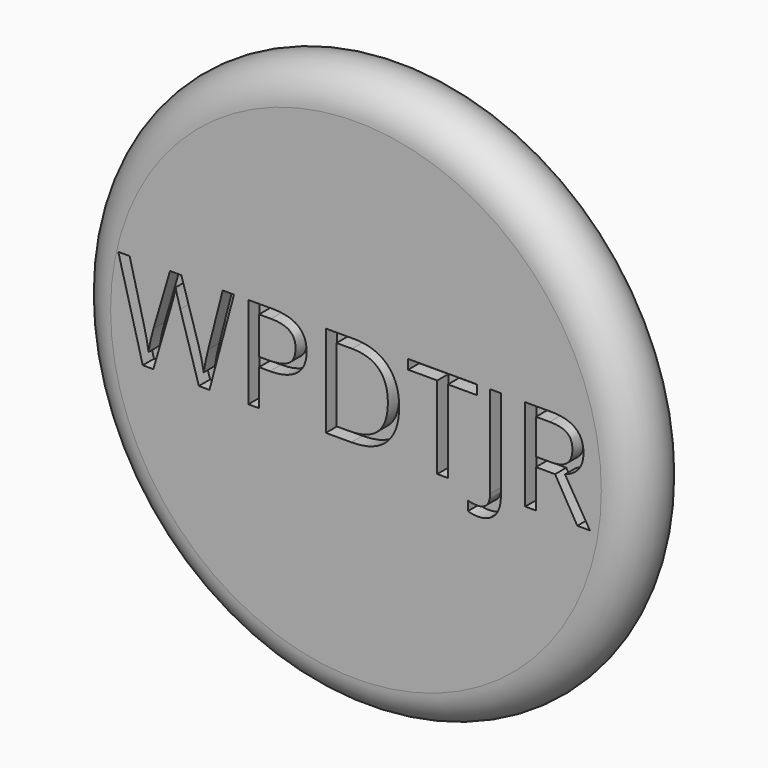
from build123d import *

# Parameters (mm, degrees)
F2_TEXT_SIZE = 23.3106116034
F3_DEPTH     = 2.54


# Not quite as in the source:
# - Text() gives the source's letters only with a copy of the font that has no kerning and outlines rounded to 1/6400 em; it was checked with that copy


with BuildPart() as f1:
    # F0 (on Top) → F1 (revolve)
    with BuildSketch(Plane.XY):
        with BuildLine():
            Line((0, 12.7), (-44.45, 12.7))
            ThreePointArc((-44.45, 12.7), (-50.8, 6.35), (-44.45, 0))
            Line((-44.45, 0), (0, 0))
            Line((0, 0), (0, 12.7))
        make_face()
    revolve(axis=Axis((0, 6.35, 0), (0, -1, 0)))

    # F2 (on face) → F3 (cut)
    with BuildSketch(Plane.XZ):
        with Locations((-43.3573805566, -6.9887411068)):
            Text('WPDTJR', F2_TEXT_SIZE, font='Open Sans', text_align=(TextAlign.LEFT, TextAlign.BOTTOM))
    extrude(amount=-F3_DEPTH, mode=Mode.SUBTRACT)


solid = f1.part
